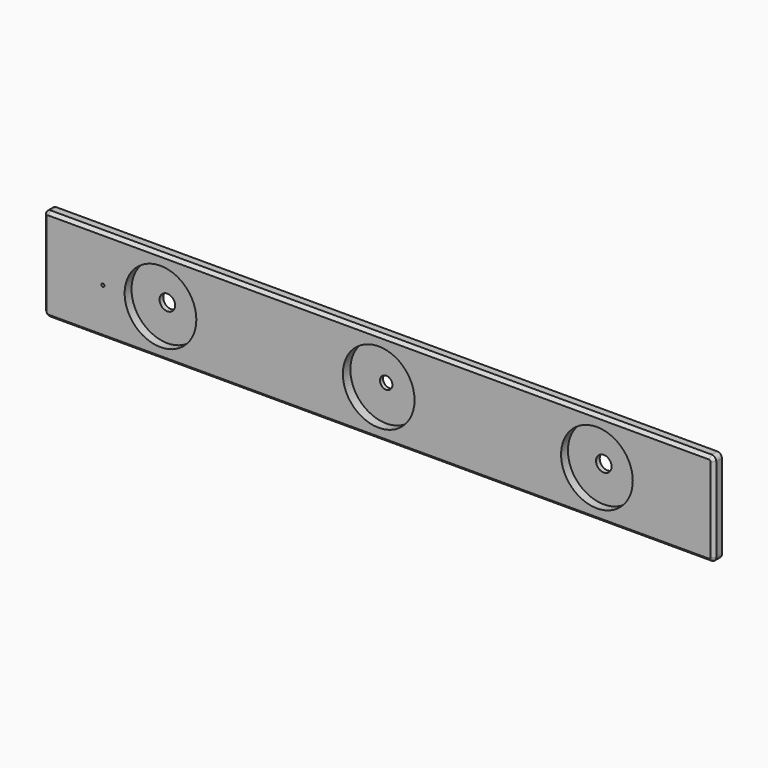
from build123d import *

# Parameters (mm, degrees)
F1_DEPTH        = 215
F0_W            = 7
F0_H            = 48
F2_DEPTH        = 202
F4_D            = 8
F4_CBORE_D      = 46
F4_CBORE_DEPTH  = 6
F5_D            = 10
F5_CBORE_D      = 46
F5_CBORE_DEPTH  = 5.5
F9_D            = 2.6
F9_DEPTH        = 8
F9_TIP          = 0.7811188047
F9_ON_F6_D      = 2.6
F9_ON_F6_DEPTH  = 8
F9_ON_F6_TIP    = 0.7811188047
F9_ON_F7_D      = 2.6
F9_ON_F7_DEPTH  = 8
F9_ON_F7_TIP    = 0.7811188047
F10_R           = 3
F11_SIZE        = 2
F14_D           = 2.6
F14_DEPTH       = 8
F14_TIP         = 0.7811188047
F15_D           = 8
F15_DEPTH       = 14
F15_CBORE_D     = 30
F15_CBORE_DEPTH = 5
F15_TIP         = 2.4034424761
F17_D           = 2
F19_D           = 5
F19_DEPTH       = 10
F19_TIP         = 1.5021515476


# Not quite as in the source:
# - a feature names something its author has since deleted; it is built from what else it names


with BuildPart() as f1:
    # F0 (on Right) → F1 (new body, symmetric)
    with BuildSketch(Plane.YZ):
        Polygon((0, 24), (0, 30), (-6.5, 30), (-6.5, 17.6169319153), (-6.5, -16.0151308179), (-6.5, -17.6169319153), (-6.5, -30), (0, -30), (0, -24), align=None)
    extrude(amount=F1_DEPTH, both=True)

    # F0 (on Right) → F2 (join, symmetric)
    with BuildSketch(Plane.YZ):
        Polygon((0, 24), (0, 30), (-6.5, 30), (-6.5, 17.6169319153), (-6.5, -16.0151308179), (-6.5, -17.6169319153), (-6.5, -30), (0, -30), (0, -24), align=None)
        with Locations((3.5, 0)):
            Rectangle(F0_W, F0_H)
    extrude(amount=F2_DEPTH, both=True)

    # F4 (through all)
    with Locations(Plane.XZ.offset(6.5)):
        with Locations((0, 0)):
            CounterBoreHole(F4_D / 2, F4_CBORE_D / 2, F4_CBORE_DEPTH)

    # F5 (through all)
    with Locations(Plane.XZ.offset(6.5)):
        with Locations((140, 0), (-140, 0)):
            CounterBoreHole(F5_D / 2, F5_CBORE_D / 2, F5_CBORE_DEPTH)

    # F9
    with Locations(Plane(origin=(-202, 0, 0), x_dir=(0, -1, 0), z_dir=(-1, 0, 0))):
        with Locations((-4, 14), (-4, -14)):
            Hole(F9_D / 2, depth=F9_DEPTH)
            with Locations((0, 0, -(F9_DEPTH + F9_TIP / 2))):  # 118° drill point
                Cone(0, F9_D / 2, F9_TIP, mode=Mode.SUBTRACT)

    # F9 on F6
    with Locations(Plane(origin=(0, 0, -24), x_dir=(1, 0, 0), z_dir=(0, 0, -1))):
        with Locations((-170, -4), (0, -4), (170, -4)):
            Hole(F9_ON_F6_D / 2, depth=F9_ON_F6_DEPTH)
            with Locations((0, 0, -(F9_ON_F6_DEPTH + F9_ON_F6_TIP / 2))):  # 118° drill point
                Cone(0, F9_ON_F6_D / 2, F9_ON_F6_TIP, mode=Mode.SUBTRACT)

    # F9 on F7
    with Locations(Plane.YZ.offset(202)):
        with Locations((4.5, -14), (4.5, 14)):
            Hole(F9_ON_F7_D / 2, depth=F9_ON_F7_DEPTH)
            with Locations((0, 0, -(F9_ON_F7_DEPTH + F9_ON_F7_TIP / 2))):  # 118° drill point
                Cone(0, F9_ON_F7_D / 2, F9_ON_F7_TIP, mode=Mode.SUBTRACT)

    # F10
    f10_edges = [f1.edges().sort_by_distance(p)[0] for p in [
        (215, -3.25, -30),
        (-215, -3.25, -30),
        (215, -3.25, 30),
        (-215, -3.25, 30),
    ]]
    fillet(f10_edges, radius=F10_R)

    # F11
    f11_edges = [f1.edges().sort_by_distance(p)[0] for p in [
        (-215, -6.5, 0),
        (0, -6.5, -30),
        (215, -6.5, 0),
        (0, -6.5, 30),
    ]]
    chamfer(f11_edges, length=F11_SIZE)

    # F14
    with Locations(Plane.XY.offset(24)):
        with Locations((0, 4), (-170, 4), (170, 4)):
            Hole(F14_D / 2, depth=F14_DEPTH)
            with Locations((0, 0, -(F14_DEPTH + F14_TIP / 2))):  # 118° drill point
                Cone(0, F14_D / 2, F14_TIP, mode=Mode.SUBTRACT)

    # F15
    with Locations(Plane(origin=(0, 7, 0), x_dir=(-1, 0, 0), z_dir=(0, 1, 0))):
        with Locations((-140, 0), (0, 0), (140, 0)):
            CounterBoreHole(F15_D / 2, F15_CBORE_D / 2, F15_CBORE_DEPTH, depth=F15_DEPTH)
            with Locations((0, 0, -(F15_DEPTH + F15_TIP / 2))):  # 118° drill point
                Cone(0, F15_D / 2, F15_TIP, mode=Mode.SUBTRACT)

    # F17 (through all)
    with Locations(Plane(origin=(0, 7, 0), x_dir=(-1, 0, 0), z_dir=(0, 1, 0))):
        with Locations((177, 0)):
            Hole(F17_D / 2)

    # F19
    with Locations(Plane(origin=(0, 7, 0), x_dir=(-1, 0, 0), z_dir=(0, 1, 0))):
        with Locations((177, 0)):
            Hole(F19_D / 2, depth=F19_DEPTH)
            with Locations((0, 0, -(F19_DEPTH + F19_TIP / 2))):  # 118° drill point
                Cone(0, F19_D / 2, F19_TIP, mode=Mode.SUBTRACT)


solid = f1.part
